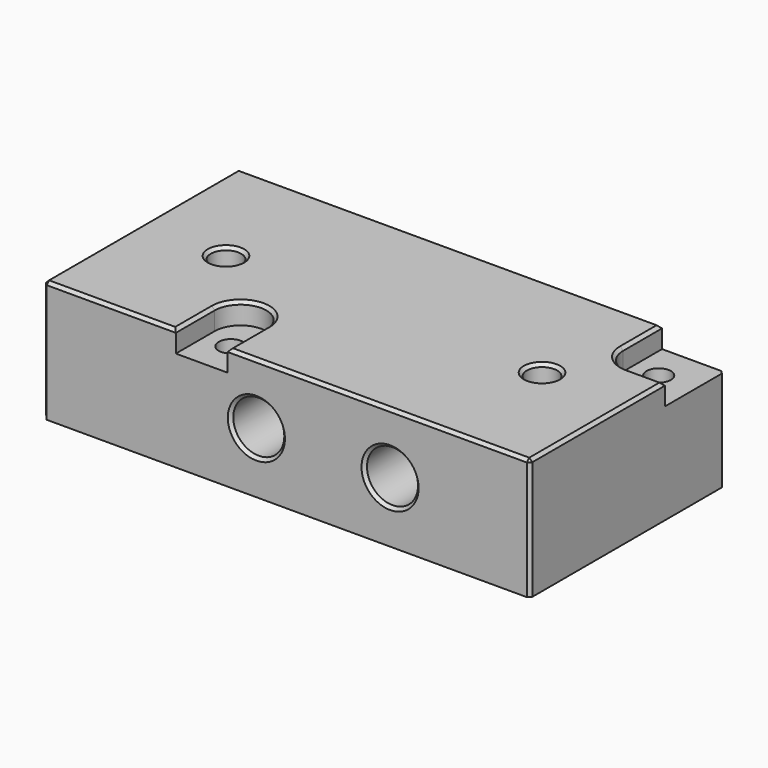
from build123d import *

# Parameters (mm, degrees)
F0_W      = 40
F0_H      = 20
F1_DEPTH  = 10
F2_R      = 2.1
F2_R_2    = 1.25
F3_DEPTH  = 5
F4_R      = 1
F6_DEPTH  = 25
F8_DEPTH  = 7
F10_DEPTH = 1.75
F9_R      = 2.1
F9_R_2    = 1.25
F11_DEPTH = 23
F12_R     = 1.25
F13_DEPTH = 5
F14_SIZE  = 0.25
F15_DEPTH = 30
F16_DEPTH = 16


# Not quite as in the source:
# - a feature names something its author has since deleted; it is built from what else it names


with BuildPart() as f1:
    # F0 (on Top) → F1 (new body)
    with BuildSketch(Plane.XY):
        with Locations((20, -10)):
            Rectangle(F0_W, F0_H)
    extrude(amount=F1_DEPTH)

    # F2 (on face) → F3 (cut)
    with BuildSketch(Plane.XZ.offset(20)):
        with Locations((28.5, 5)):
            Circle(F2_R)
        with Locations((28.5, 5)):
            Circle(F2_R_2, mode=Mode.SUBTRACT)
        with Locations((17.5, 5)):
            Circle(F2_R)
        with Locations((17.5, 5)):
            Circle(F2_R_2, mode=Mode.SUBTRACT)
    extrude(amount=-F3_DEPTH, mode=Mode.SUBTRACT)

    # F4 (on face) → F6 (cut)
    with BuildSketch(Plane.XY.offset(10)):
        with Locations((13, -17)):
            Circle(F4_R)
        with Locations((37, -3)):
            Circle(F4_R)
    extrude(amount=-F6_DEPTH, mode=Mode.SUBTRACT)

    # F7 (on face) → F8 (cut)
    with BuildSketch(Plane(origin=(0, 0, 0), x_dir=(1, 0, 0), z_dir=(0, 0, -1))):
        with BuildLine():
            Line((16.25, 11.25), (15.5, 11.25))
            ThreePointArc((15.5, 11.25), (14.25, 10), (15.5, 8.75))
            Line((15.5, 8.75), (16.25, 8.75))
            ThreePointArc((16.25, 8.75), (17.5, 10), (16.25, 11.25))
        make_face()
        with BuildLine():
            Line((27.25, 11.25), (26.5, 11.25))
            ThreePointArc((26.5, 11.25), (25.25, 10), (26.5, 8.75))
            Line((26.5, 8.75), (27.25, 8.75))
            ThreePointArc((27.25, 8.75), (28.5, 10), (27.25, 11.25))
        make_face()
    extrude(amount=-F8_DEPTH, mode=Mode.SUBTRACT)

    # F4 (on face) → F10 (cut)
    with BuildSketch(Plane.XY.offset(10)):
        with BuildLine():
            Line((15.125, -20), (15.125, -16))
            ThreePointArc((15.125, -16), (13, -13.875), (10.875, -16))
            Line((10.875, -16), (10.875, -20))
            Line((10.875, -20), (15.125, -20))
        make_face()
        with Locations((13, -17)):
            Circle(F4_R, mode=Mode.SUBTRACT)
        with BuildLine():
            Line((37, -6.125), (40, -6.125))
            Line((40, -6.125), (40, 0))
            Line((40, 0), (34.875, 0))
            Line((34.875, 0), (34.875, -4))
            ThreePointArc((34.875, -4), (35.49739809, -5.50260191), (37, -6.125))
        make_face()
        with Locations((37, -3)):
            Circle(F4_R, mode=Mode.SUBTRACT)
    extrude(amount=-F10_DEPTH, mode=Mode.SUBTRACT)

    # F9 (on face) → F11 (cut)
    with BuildSketch(Plane(origin=(0, 0, 0), x_dir=(0, -1, 0), z_dir=(-1, 0, 0))):
        with Locations((5, 5)):
            Circle(F9_R)
        with Locations((5, 5)):
            Circle(F9_R_2, mode=Mode.SUBTRACT)
    extrude(amount=-F11_DEPTH, mode=Mode.SUBTRACT)

    # F12 (on face) → F13 (cut)
    with BuildSketch(Plane.XY.offset(10)):
        with Locations((7, -10)):
            Circle(F12_R)
        with Locations((33, -10)):
            Circle(F12_R)
    extrude(amount=-F13_DEPTH, mode=Mode.SUBTRACT)

    # F14
    f14_edges = [f1.edges().sort_by_distance(p)[0] for p in [
        (15.4, -20, 5),
        (26.4, -20, 5),
        (0, 0, 5),
        (0, -20, 5),
        (34.875, -2, 10),
        (17.4375, 0, 10),
        (35.497398, -5.502602, 10),
        (0, -10, 10),
        (38.5, -6.125, 10),
        (5.4375, -20, 10),
        (40, -13.0625, 10),
        (10.875, -18, 10),
        (27.5625, -20, 10),
        (13, -13.875, 10),
        (15.125, -18, 10),
        (5.75, -10, 10),
        (31.75, -10, 10),
        (0, -10, 0),
        (40, -20, 5),
        (40, 0, 4.125),
        (0, -2.9, 5),
    ]]
    chamfer(f14_edges, length=F14_SIZE)

    # F15 (cut): a face of the model
    f15_faces = [f1.faces().sort_by_distance(p)[0] for p in [
        (0, -5, 5),
    ]]
    extrude(f15_faces, amount=-F15_DEPTH, mode=Mode.SUBTRACT)

    # F16 (cut): faces of the model
    f16_faces = [f1.faces().sort_by_distance(p)[0] for p in [
        (17.5, -20, 5),
        (28.5, -20, 5),
    ]]
    extrude(f16_faces, amount=-F16_DEPTH, mode=Mode.SUBTRACT)


solid = f1.part
